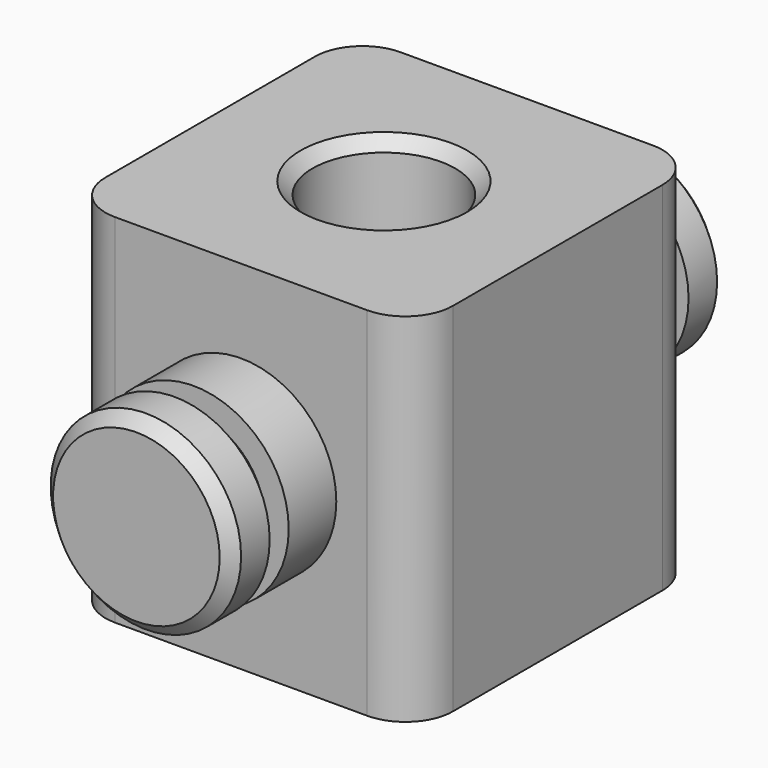
from build123d import *

# Parameters (mm, degrees)
F0_R     = 3
F1_DEPTH = 7.5
F2_SIZE2 = 0.5
F2_SIZE  = 0.5
F3_R     = 4
F4_DEPTH = 5.5
F5_SIZE2 = 0.5
F5_SIZE  = 0.5
F6_W     = 1
F6_H     = 1


# Not quite as in the source:
# - a feature of the source that left no trace in its solid (it failed there, or was rolled back) is left out
# - a pattern or mirror of a feature is missing from the dataset's text; its kind, count and spacing are read off the source's solid


with BuildPart() as f1:
    # F0 (on Top) → F1 (new body, symmetric)
    with BuildSketch(Plane.XY):
        with BuildLine():
            ThreePointArc((7.3, 5.5), (6.7142135624, 6.9142135624), (5.3, 7.5))
            Line((5.3, 7.5), (-5.3, 7.5))
            ThreePointArc((-5.3, 7.5), (-6.7142135624, 6.9142135624), (-7.3, 5.5))
            Line((-7.3, 5.5), (-7.3, -5.5))
            ThreePointArc((-7.3, -5.5), (-6.7142135624, -6.9142135624), (-5.3, -7.5))
            Line((-5.3, -7.5), (5.3, -7.5))
            ThreePointArc((5.3, -7.5), (6.7142135624, -6.9142135624), (7.3, -5.5))
            Line((7.3, -5.5), (7.3, 5.5))
        make_face()
        Circle(F0_R, mode=Mode.SUBTRACT)
    extrude(amount=F1_DEPTH, both=True)

    # F2
    f2_edges = [f1.edges().sort_by_distance(p)[0] for p in [
        (-3, 0, 7.5),
        (-3, 0, -7.5),
    ]]
    chamfer(f2_edges, length=F2_SIZE, length2=F2_SIZE2)

    # F3 (on face) → F4 (join)
    with BuildSketch(Plane.XZ.offset(7.5)):
        Circle(F3_R)
    f4 = extrude(amount=F4_DEPTH)

    # F4_copies: F4 across plane
    add(f4.mirror(Plane.ZX))

    # F5
    f5_edges = [f1.edges().sort_by_distance(p)[0] for p in [
        (-4, -13, 0),
        (-4, 13, 0),
    ]]
    chamfer(f5_edges, length=F5_SIZE, length2=F5_SIZE2)

    # F6 (on Right) → F7 (revolve, cut)
    with BuildSketch(Plane.YZ):
        with Locations((-10.5, 3.5)):
            Rectangle(F6_W, F6_H)
    f7 = revolve(axis=Axis((0, -13, 0), (0, -1, 0)), mode=Mode.SUBTRACT)

    # F7_copies: F7 across plane
    add(f7.mirror(Plane.ZX), mode=Mode.SUBTRACT)


solid = f1.part
